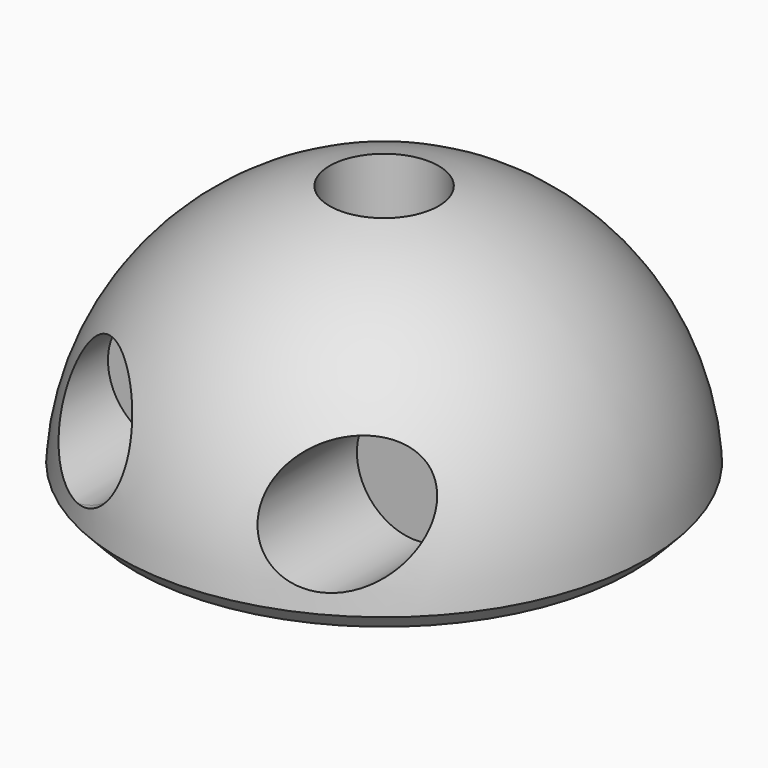
from build123d import *

# Parameters (mm, degrees)
F3_R      = 3.75
F4_DEPTH  = 7.5
F6_R      = 2.25
F7_DEPTH  = 17.001
F9_R      = 3.5
F10_DEPTH = 25


# Not quite as in the source:
# - a fillet or chamfer that OpenCascade refuses, or shapes differently, is made with other operations: its cross-section is extruded or revolved along the edge and cut away or added


with BuildPart() as f1:
    # F0 (on Front) → F1 (revolve)
    with BuildSketch(Plane.XZ):
        with BuildLine():
            Line((0, 0), (17, 0))
            ThreePointArc((17, 0), (12.0208152802, 12.0208152802), (0, 17))
            Line((0, 17), (0, 0))
        make_face()
    revolve(axis=Axis((0, 0, 8.5), (0, 0, 1)))

    # F3 (on offset) → F4 (cut, symmetric)
    with BuildSketch(Plane.XZ.offset(15)):
        with Locations((-8, 6)):
            Circle(F3_R)
        with Locations((8, 6)):
            Circle(F3_R)
    extrude(amount=F4_DEPTH, both=True, mode=Mode.SUBTRACT)

    # F5: chamfer of 1 on 1 edges, made by hand

    # F5_s1 → F5_t2 (revolve, cut)
    with BuildSketch(Plane.XZ):
        with BuildLine():
            Line((15.9687194227, 0), (16.9667643866, 1.0625))
            ThreePointArc((16.9667643866, 1.0625), (16.9912411836, 0.54564003), (17, 0))
            Line((17, 0), (15.9687194227, 0))
        make_face()
    revolve(axis=Axis((0, 0, 0), (0, 0, 1)), mode=Mode.SUBTRACT)

    # F6 (on Top) → F7 (cut, through all)
    with BuildSketch(Plane.XY):
        Circle(F6_R)
    extrude(amount=F7_DEPTH, mode=Mode.SUBTRACT)

    # F9 (on offset) → F10 (cut)
    with BuildSketch(Plane.XY.offset(30)):
        Circle(F9_R)
    extrude(amount=-F10_DEPTH, mode=Mode.SUBTRACT)


solid = f1.part
